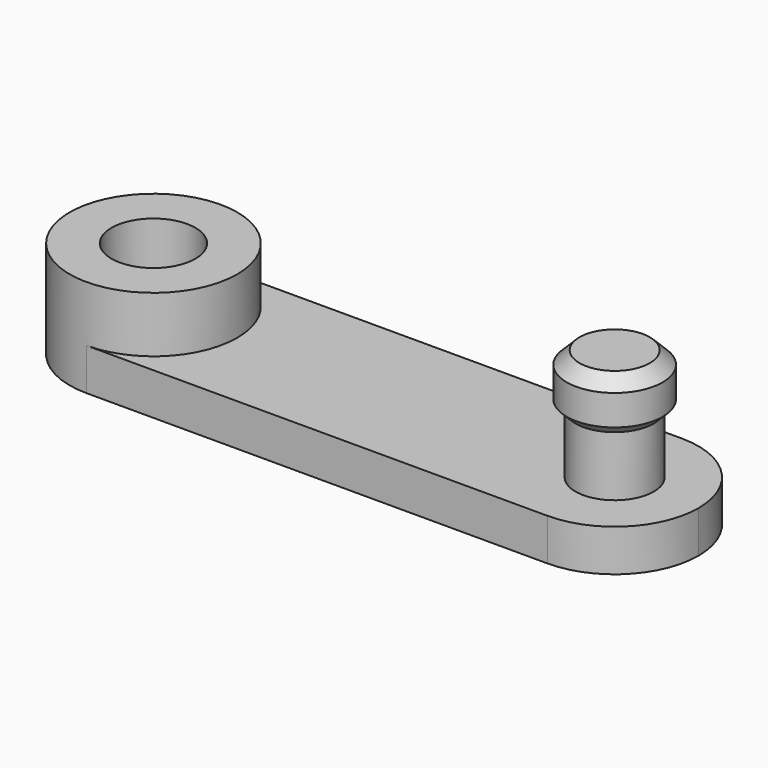
from build123d import *

# Parameters (mm, degrees)
F1_DEPTH    = 1.5
F2_R        = 1.4
F3_DEPTH    = 4
F4_R        = 1.7145
F5_DEPTH    = 2
F6_SIZE     = 0.4572
F7_S5_R     = 1.4
F7_T6_DEPTH = 4
F8_R        = 3
F9_DEPTH    = 2
F10_DEPTH   = 25.4


# Not quite as in the source:
# - a fillet or chamfer that OpenCascade refuses, or shapes differently, is made with other operations: its cross-section is extruded or revolved along the edge and cut away or added


with BuildPart() as f1:
    # F0 (on Top) → F1 (new body)
    with BuildSketch(Plane.XY):
        with BuildLine():
            Line((-9.5, -3), (7, -3))
            ThreePointArc((7, -3), (4, 0), (7, 3))
            Line((7, 3), (-9.5, 3))
            ThreePointArc((-9.5, 3), (-7.3786796564, 2.1213203436), (-6.5, 0))
            ThreePointArc((-6.5, 0), (-7.3786796564, -2.1213203436), (-9.5, -3))
        make_face()
        with BuildLine():
            ThreePointArc((7, 3), (4, 0), (7, -3))
            ThreePointArc((7, -3), (9.1213203436, -2.1213203436), (10, 0))
            ThreePointArc((10, 0), (9.1213203436, 2.1213203436), (7, 3))
        make_face()
        with BuildLine():
            ThreePointArc((-9.5, 3), (-12.5, 0), (-9.5, -3))
            Line((-9.5, -3), (-9.5, -1.5))
            ThreePointArc((-9.5, -1.5), (-11, 0), (-9.5, 1.5))
            Line((-9.5, 1.5), (-9.5, 3))
        make_face()
        with BuildLine():
            Line((-9.5, -1.5), (-9.5, -3))
            ThreePointArc((-9.5, -3), (-7.3786796564, -2.1213203436), (-6.5, 0))
            ThreePointArc((-6.5, 0), (-7.3786796564, 2.1213203436), (-9.5, 3))
            Line((-9.5, 3), (-9.5, 1.5))
            ThreePointArc((-9.5, 1.5), (-8.4393398282, 1.0606601718), (-8, 0))
            ThreePointArc((-8, 0), (-8.4393398282, -1.0606601718), (-9.5, -1.5))
        make_face()
    extrude(amount=F1_DEPTH)

    # F2 (on face) → F3 (join)
    with BuildSketch(Plane.XY.offset(1.5)):
        with Locations((7, 0)):
            Circle(F2_R)
    extrude(amount=F3_DEPTH)

    # F4 (on face) → F5 (join)
    with BuildSketch(Plane.XY.offset(5.5)):
        with Locations((7, 0)):
            Circle(F4_R)
    extrude(amount=-F5_DEPTH)

    # F6
    f6_edges = [f1.edges().sort_by_distance(p)[0] for p in [
        (5.2855, 0, 5.5),
    ]]
    chamfer(f6_edges, length=F6_SIZE)

    # F7: chamfer of 0.4572 on 1 edges, made by hand


with BuildPart() as f7_tool2:
    # F7_s3 → F7_t4 (revolve)
    with BuildSketch(Plane.XZ):
        Polygon((8.7145, 3.9572), (8.2573, 3.5), (8.7145, 3.5), align=None)
    revolve(axis=Axis((7, 0, 3.5), (0, 0, 1)))

    # F7_s5 → F7_t6 (cut, symmetric)
    with BuildSketch(Plane.XY.offset(3.7)):
        with Locations((7, 0)):
            Circle(F7_S5_R)
    extrude(amount=F7_T6_DEPTH, both=True, mode=Mode.SUBTRACT)


with BuildPart() as f1_1:
    add(f1.part)

    # F7_t1: cut F7_tool2
    add(f7_tool2.part, mode=Mode.SUBTRACT)

    # F8 (on face) → F9 (join)
    with BuildSketch(Plane.XY.offset(1.5)):
        with Locations((-9.5, 0)):
            Circle(F8_R)
    extrude(amount=F9_DEPTH)

    # F10 (cut): a face of the model
    f10_faces = [f1_1.faces().sort_by_distance(p)[0] for p in [
        (-9.5, 0, 1.5),
    ]]
    extrude(f10_faces, amount=-F10_DEPTH, mode=Mode.SUBTRACT)


solid = f1_1.part
